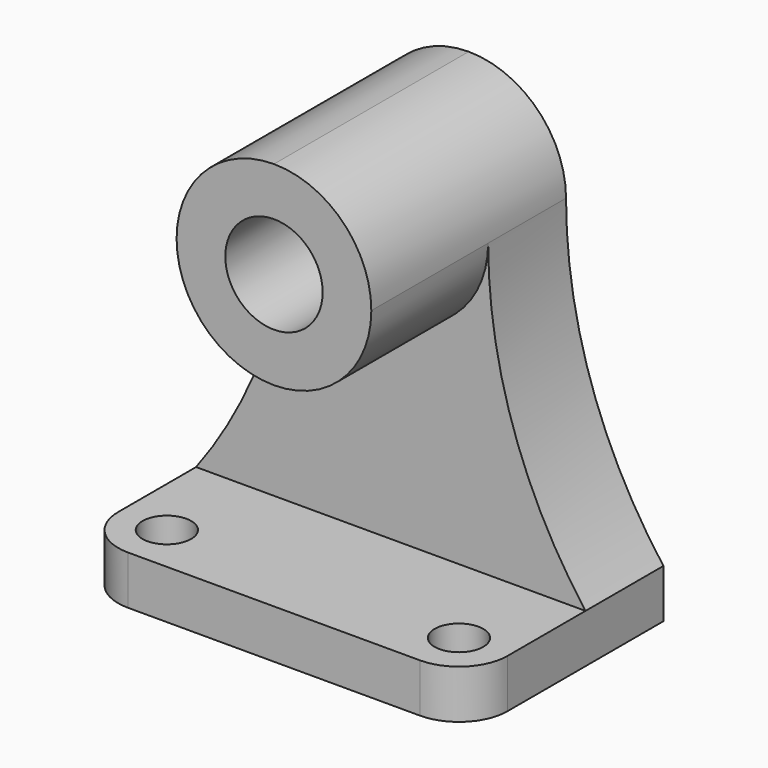
from build123d import *

# Parameters (mm, degrees)
F1_DEPTH  = 31.75
F3_DEPTH  = 31.75
F7_DEPTH  = 19.05
F9_W      = 50.8
F9_H      = 19.05
F10_DEPTH = 31.75
F11_DEPTH = 19.05
F13_DEPTH = 19.05
F14_DEPTH = 12.7
F15_DEPTH = 12.7
F17_DEPTH = 12.7
F18_R     = 6.35
F19_DEPTH = 31.75
F20_R     = 3.175
F21_DEPTH = 6.35
F23_DEPTH = 6.35
F25_DEPTH = 6.35


with BuildPart() as f1:
    # F0 (on Front) → F1 (new body)
    with BuildSketch(Plane.XZ):
        Polygon((0, 6.35), (0, 0), (50.8, 0), (50.8, 6.35), (38.1, 6.35), (38.1, 57.15), (12.7, 57.15), (12.7, 6.35), align=None)
    extrude(amount=F1_DEPTH)

    # F2 (on face) → F3 (cut)
    with BuildSketch(Plane.XZ.offset(31.75)):
        with BuildLine():
            ThreePointArc((12.7, 44.45), (16.4197438789, 53.4302561211), (25.4, 57.15))
            Line((25.4, 57.15), (12.7, 57.15))
            Line((12.7, 57.15), (12.7, 44.45))
        make_face()
        with BuildLine():
            ThreePointArc((25.4, 57.15), (34.3802561211, 53.4302561211), (38.1, 44.45))
            Line((38.1, 44.45), (38.1, 57.15))
            Line((38.1, 57.15), (25.4, 57.15))
        make_face()
    extrude(amount=-F3_DEPTH, mode=Mode.SUBTRACT)

    # F5 (on face) → F7 (cut)
    with BuildSketch(Plane.XZ.offset(31.75)):
        with BuildLine():
            ThreePointArc((38.1, 44.45), (34.3802561211, 35.4697438789), (25.4, 31.75))
            Line((25.4, 31.75), (38.1, 31.75))
            Line((38.1, 31.75), (38.1, 44.45))
        make_face()
    extrude(amount=-F7_DEPTH, mode=Mode.SUBTRACT)

    # F9 (on face) → F10 (cut)
    with BuildSketch(Plane(origin=(0, 0, 0), x_dir=(1, 0, 0), z_dir=(0, 0, -1))):
        with Locations((25.4, 22.225)):
            Rectangle(F9_W, F9_H)
    extrude(amount=-F10_DEPTH, mode=Mode.SUBTRACT)

    # F8 (on face) → F11 (cut)
    with BuildSketch(Plane.XZ.offset(31.75)):
        with BuildLine():
            Line((12.7, 31.75), (25.4, 31.75))
            ThreePointArc((25.4, 31.75), (16.4197438789, 35.4697438789), (12.7, 44.45))
            Line((12.7, 44.45), (12.7, 31.75))
        make_face()
    extrude(amount=-F11_DEPTH, mode=Mode.SUBTRACT)

    # F12 (on face) → F13 (join)
    with BuildSketch(Plane.XZ.offset(12.7)):
        Polygon((38.1, 6.35), (12.7, 6.35), (0, 6.35), (0, 0), (50.8, 0), (50.8, 6.35), align=None)
    extrude(amount=F13_DEPTH)

    # F14 (add): a face of the model
    f14_faces = [f1.faces().sort_by_distance(p)[0] for p in [
        (12.7, -6.35, 25.4),
    ]]
    extrude(f14_faces, amount=F14_DEPTH)

    # F15 (add): a face of the model
    f15_faces = [f1.faces().sort_by_distance(p)[0] for p in [
        (38.1, -6.35, 25.4),
    ]]
    extrude(f15_faces, amount=F15_DEPTH)

    # F16 (on face) → F17 (cut)
    with BuildSketch(Plane.XZ.offset(12.7)):
        with BuildLine():
            Line((0, 44.45), (0, 6.35))
            ThreePointArc((0, 6.35), (9.4413894262, 24.3695368579), (12.7, 44.45))
            Line((12.7, 44.45), (0, 44.45))
        make_face()
        with BuildLine():
            ThreePointArc((38.1, 44.45), (41.3586105738, 24.3695368579), (50.8, 6.35))
            Line((50.8, 6.35), (50.8, 44.45))
            Line((50.8, 44.45), (38.1, 44.45))
        make_face()
    extrude(amount=-F17_DEPTH, mode=Mode.SUBTRACT)

    # F18 (on face) → F19 (cut)
    with BuildSketch(Plane.XZ.offset(31.75)):
        with Locations((25.4, 44.4756895304)):
            Circle(F18_R)
    extrude(amount=-F19_DEPTH, mode=Mode.SUBTRACT)

    # F20 (on face) → F21 (cut)
    with BuildSketch(Plane.XY.offset(6.35)):
        with Locations((44.45, -25.4)):
            Circle(F20_R)
        with Locations((6.35, -25.4)):
            Circle(F20_R)
    extrude(amount=-F21_DEPTH, mode=Mode.SUBTRACT)

    # F22 (on face) → F23 (cut)
    with BuildSketch(Plane.XY.offset(6.35)):
        with BuildLine():
            ThreePointArc((6.35, -31.75), (1.8598719395, -29.8901280605), (0, -25.4))
            Line((0, -25.4), (0, -31.75))
            Line((0, -31.75), (6.35, -31.75))
        make_face()
    extrude(amount=-F23_DEPTH, mode=Mode.SUBTRACT)

    # F24 (on face) → F25 (cut)
    with BuildSketch(Plane.XY.offset(6.35)):
        with BuildLine():
            ThreePointArc((50.8, -25.4), (48.9401280605, -29.8901280605), (44.45, -31.75))
            Line((44.45, -31.75), (50.8, -31.75))
            Line((50.8, -31.75), (50.8, -25.4))
        make_face()
    extrude(amount=-F25_DEPTH, mode=Mode.SUBTRACT)


solid = f1.part
